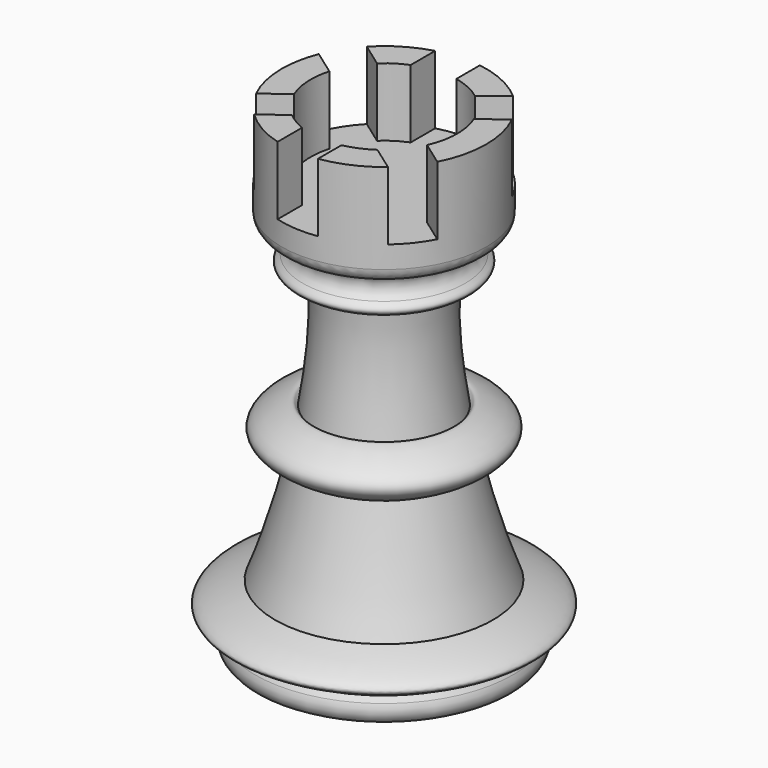
from build123d import *

# Parameters (mm, degrees)
F2_R     = 1.27
F4_DEPTH = 6.35


with BuildPart() as f1:
    # F0 (on Front) → F1 (revolve)
    with BuildSketch(Plane.XZ):
        with BuildLine():
            add(Edge.make_bspline(
                [(-28.4966456652, -6.8399562779), (-29.3284551449, -8.3585751384), (-30.1182179448, -9.2634102158), (-30.770753986, -9.2634102158)],
                knots=[29.675354213, 29.675354213, 29.675354213, 29.675354213, 35.171877189, 35.171877189, 35.171877189, 35.171877189], degree=3))
            Line((-30.770753986, -9.2634102158), (-16.800753986, -9.2634102158))
            Line((-16.800753986, -9.2634102158), (-16.800753986, 35.3643707931))
            Line((-16.800753986, 35.3643707931), (-26.325753986, 35.3643707931))
            Line((-26.325753986, 35.3643707931), (-26.325753986, 25.6264582276))
            add(Edge.make_bspline(
                [(-26.325753986, 25.6264582276), (-24.8220720213, 25.9674204899), (-23.7998688188, 25.3312059181), (-23.1610279839, 24.0178447701)],
                knots=[0, 0, 0, 0, 5.552474267, 5.552474267, 5.552474267, 5.552474267], degree=3))
            add(Edge.make_bspline(
                [(-23.1610279839, 24.0178447701), (-22.8370089862, 23.3517102033), (-22.6116100093, 22.5113795883), (-22.4720291366, 21.535999924)],
                knots=[5.552474267, 5.552474267, 5.552474267, 5.552474267, 8.3686798828, 8.3686798828, 8.3686798828, 8.3686798828], degree=3))
            add(Edge.make_bspline(
                [(-22.4720291366, 21.535999924), (-22.0770253148, 18.7757456898), (-22.3692951404, 14.9339521497), (-23.0587029188, 10.8978256431)],
                knots=[8.3686798828, 8.3686798828, 8.3686798828, 8.3686798828, 16.3383390414, 16.3383390414, 16.3383390414, 16.3383390414], degree=3))
            add(Edge.make_bspline(
                [(-23.0587029188, 10.8978256431), (-23.2933772487, 9.5239286357), (-23.5740687806, 8.1275138626), (-23.8893337374, 6.7435752652)],
                knots=[16.3383390414, 16.3383390414, 16.3383390414, 16.3383390414, 19.0512101196, 19.0512101196, 19.0512101196, 19.0512101196], degree=3))
            add(Edge.make_bspline(
                [(-23.8893337374, 6.7435752652), (-24.7332275919, 3.0390808319), (-25.8248446305, -0.5760201452), (-26.9446993916, -3.4305627711)],
                knots=[19.0512101196, 19.0512101196, 19.0512101196, 19.0512101196, 26.312959901, 26.312959901, 26.312959901, 26.312959901], degree=3))
            add(Edge.make_bspline(
                [(-26.9446993916, -3.4305627711), (-27.4632236305, -4.752296262), (-27.9878018969, -5.9109698185), (-28.4966456652, -6.8399562779)],
                knots=[26.312959901, 26.312959901, 26.312959901, 26.312959901, 29.675354213, 29.675354213, 29.675354213, 29.675354213], degree=3))
        make_face()
        with BuildLine():
            add(Edge.make_bspline(
                [(-28.4966456652, -6.8399562779), (-29.4493708837, -6.1436897859), (-32.4468383476, -5.4496032834), (-28.6449505836, -3.8868749556), (-26.9446993916, -3.4305627711)],
                knots=[0, 0, 0, 0, 0.4432086015, 1, 1, 1, 1], degree=3))
            add(Edge.make_bspline(
                [(-26.9446993916, -3.4305627711), (-27.4632236305, -4.752296262), (-27.9878018969, -5.9109698185), (-28.4966456652, -6.8399562779)],
                knots=[26.312959901, 26.312959901, 26.312959901, 26.312959901, 29.675354213, 29.675354213, 29.675354213, 29.675354213], degree=3))
        make_face()
        with BuildLine():
            add(Edge.make_bspline(
                [(-23.8893337374, 6.7435752652), (-25.8194649176, 7.6878634155), (-28.4616478332, 9.2987396297), (-23.3220318401, 11.7928811589), (-23.2745634428, 11.1261067843), (-23.0587029188, 10.8978256431)],
                knots=[0, 0, 0, 0, 0.4194167532, 0.826524063, 1, 1, 1, 1], degree=3))
            add(Edge.make_bspline(
                [(-23.0587029188, 10.8978256431), (-23.2933772487, 9.5239286357), (-23.5740687806, 8.1275138626), (-23.8893337374, 6.7435752652)],
                knots=[16.3383390414, 16.3383390414, 16.3383390414, 16.3383390414, 19.0512101196, 19.0512101196, 19.0512101196, 19.0512101196], degree=3))
        make_face()
        with BuildLine():
            add(Edge.make_bspline(
                [(-23.1610279839, 24.0178447701), (-22.8370089862, 23.3517102033), (-22.6116100093, 22.5113795883), (-22.4720291366, 21.535999924)],
                knots=[5.552474267, 5.552474267, 5.552474267, 5.552474267, 8.3686798828, 8.3686798828, 8.3686798828, 8.3686798828], degree=3))
            add(Edge.make_bspline(
                [(-23.1610279839, 24.0178447701), (-24.0927796522, 23.5327420351), (-25.7238369486, 22.6368880839), (-23.7519857815, 21.8821803215), (-22.4720291366, 21.535999924)],
                knots=[0, 0, 0, 0, 0.4724642692, 1, 1, 1, 1], degree=3))
        make_face()
    revolve(axis=Axis((-16.800753986, 0, 13.0504802887), (0, 0, -1)))

    # F2
    f2_edges = [f1.edges().sort_by_distance(p)[0] for p in [
        (-2.830754, 0, -9.26341),
        (-7.275754, 0, 25.626458),
        (-10.44048, 0, 24.017845),
    ]]
    fillet(f2_edges, radius=F2_R)

    # F3 (on face) → F4 (cut)
    with BuildSketch(Plane.XY.offset(35.3643707931)):
        with BuildLine():
            ThreePointArc((-15.4147866141, 9.4236255997), (-17.4069571494, 9.5056900183), (-19.3725646564, 9.1712275555))
            Line((-19.3725646564, 9.1712275555), (-19.3725646564, 6.32408119))
            ThreePointArc((-19.3725646564, 6.32408119), (-20.472143023, 5.7557897426), (-21.4510415881, 4.9983035362))
            Line((-21.4510415881, 4.9983035362), (-23.6780484526, 6.5900262381))
            ThreePointArc((-23.6780484526, 6.5900262381), (-24.8218239255, 5.1369311874), (-25.6632623961, 3.4902105496))
            Line((-25.6632623961, 3.4902105496), (-23.3716803438, 1.8523336153))
            ThreePointArc((-23.3716803438, 1.8523336153), (-23.6181605612, -0.3621886379), (-23.1384280379, -2.5381293572))
            Line((-23.1384280379, -2.5381293572), (-25.3399225374, -4.2199793188))
            ThreePointArc((-25.3399225374, -4.2199793188), (-24.4898691375, -5.6216664065), (-23.4120620736, -6.8568382196))
            Line((-23.4120620736, -6.8568382196), (-21.1848628294, -5.2333357116))
            ThreePointArc((-21.1848628294, -5.2333357116), (-20.3212135434, -5.8493228263), (-19.3725646564, -6.32408119))
            Line((-19.3725646564, -6.32408119), (-19.3725646564, -9.1712275555))
            ThreePointArc((-19.3725646564, -9.1712275555), (-17.4069571494, -9.5056900183), (-15.4147866141, -9.4236255997))
            Line((-15.4147866141, -9.4236255997), (-15.4147866141, -6.6848565778))
            ThreePointArc((-15.4147866141, -6.6848565778), (-14.1142250097, -6.2762070617), (-12.9207860056, -5.6173001961))
            Line((-12.9207860056, -5.6173001961), (-10.6292039533, -7.2551771305))
            ThreePointArc((-10.6292039533, -7.2551771305), (-9.3436009035, -5.9259170517), (-8.3390792213, -4.3732922584))
            Line((-8.3390792213, -4.3732922584), (-10.5660860859, -2.7815695565))
            ThreePointArc((-10.5660860859, -2.7815695565), (-9.9746816223, -0.1137941453), (-10.4768357965, 2.5722114522))
            Line((-10.4768357965, 2.5722114522), (-8.2496365523, 4.1957139602))
            ThreePointArc((-8.2496365523, 4.1957139602), (-9.2235636356, 5.7716385364), (-10.4841293021, 7.129226999))
            Line((-10.4841293021, 7.129226999), (-12.6856238016, 5.4473770374))
            ThreePointArc((-12.6856238016, 5.4473770374), (-13.9814708353, 6.2177050057), (-15.4147866141, 6.6848565778))
            Line((-15.4147866141, 6.6848565778), (-15.4147866141, 9.4236255997))
        make_face()
    extrude(amount=-F4_DEPTH, mode=Mode.SUBTRACT)


solid = f1.part
